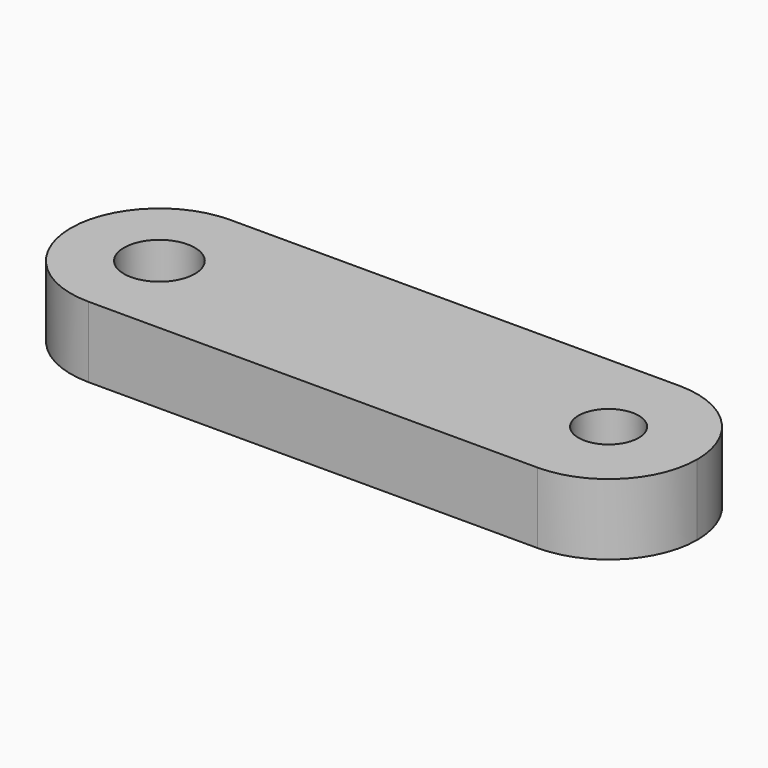
from build123d import *

# Parameters (mm, degrees)
F0_W     = 70.698
F0_H     = 20
F1_DEPTH = 8
F2_D     = 8
F3_D     = 6.8
F4_R     = 9.99999


# Not quite as in the source:
# - a fillet or chamfer is up to 0.001 mm smaller than in the source, because OpenCascade refuses the exact size


with BuildPart() as f1:
    # F0 (on Top) → F1 (new body)
    with BuildSketch(Plane.XY):
        Rectangle(F0_W, F0_H)
    extrude(amount=-F1_DEPTH)

    # F2 (through all)
    with Locations(Plane.XY):
        with Locations((-25.349, 0)):
            Hole(F2_D / 2)

    # F3 (through all)
    with Locations(Plane.XY):
        with Locations((25.349, 0)):
            Hole(F3_D / 2)

    # F4 (radius 10 in the source; OpenCascade refuses exactly that, so slightly less here)
    f4_edges = [f1.edges().sort_by_distance(p)[0] for p in [
        (35.349, 10, -4),
        (35.349, -10, -4),
        (-35.349, 10, -4),
        (-35.349, -10, -4),
    ]]
    fillet(f4_edges, radius=F4_R)


solid = f1.part
